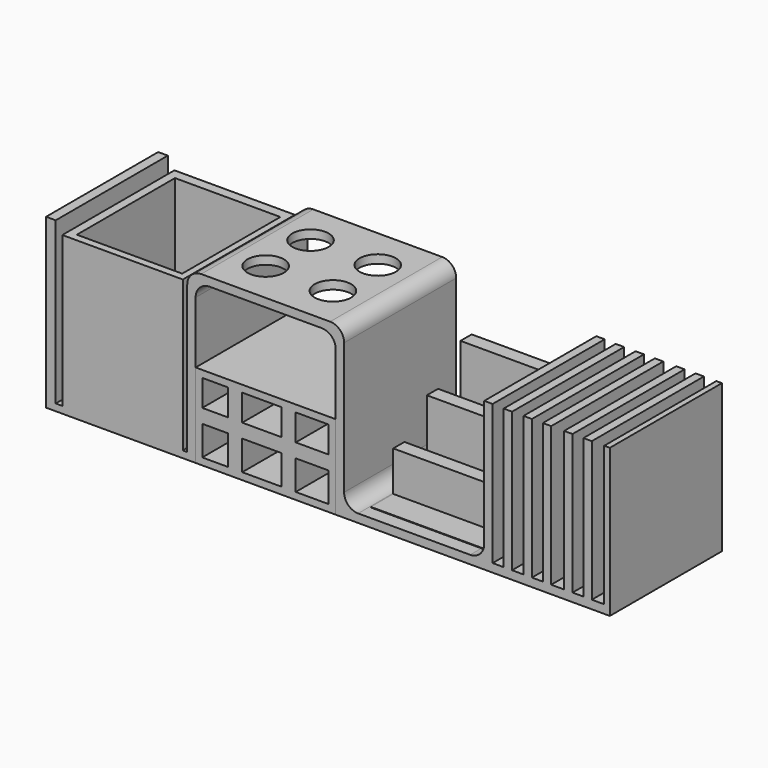
from build123d import *

# Parameters (mm, degrees)
F0_W      = 2
F0_H      = 49.8195460532
F0_W_2    = 3
F1_DEPTH  = 50
F4_W      = 40
F4_H      = 15
F5_DEPTH  = 36.1
F6_W      = 40
F6_H      = 10
F7_DEPTH  = 35.5
F8_W      = 40
F8_H      = 15
F9_DEPTH  = 25.1
F10_W     = 40
F10_H     = 10
F11_DEPTH = 24.8
F12_W     = 40
F12_H     = 15
F13_DEPTH = 14.5
F14_W     = 40
F14_H     = 10
F15_DEPTH = 14.3
F16_R     = 5
F3_W      = 50
F3_H      = 50
F17_DEPTH = 30
F18_T     = -2.5
F2_R      = 6.5
F19_DEPTH = 13.9
F20_W     = 43
F20_H     = 50
F21_DEPTH = 53.7
F22_W     = 37.6056898385
F22_H     = 43.7766639516
F23_DEPTH = 51.1
F24_W     = 9.2634954209
F24_H     = 5.0000008196
F24_W_2   = 5.0000008196
F24_H_2   = 9.4318167865
F24_W_3   = 14.0909086913
F24_H_3   = 10.5681823939
F24_W_4   = 5.0000026822
F24_W_5   = 11.6455923861
F25_DEPTH = 47.5


with BuildPart() as f1:
    # F0 (on Front) → F1 (new body)
    with BuildSketch(Plane.XZ):
        Polygon((4.5763543636, 0), (4.5763543636, 57), (54.5763543636, 57), (54.5763543636, 0), (107.5763543636, 0), (107.5763543636, 3), (57.5763543636, 3), (57.5763543636, 60), (1.5763543636, 60), (1.5763543636, 2.4467778858), (-45.3553423285, 2.4467778858), (-45.3553423285, 60), (-48.798955977, 60), (-48.798955977, 0), (-45.3553423285, 0), (1.5763543636, 0), align=None)
        Polygon((107.5763543636, 3), (107.5763543636, 0), (110.5763543636, 0), (152.4111737013, 0), (152.4111737013, 3.0127370264), (150.4111737013, 3.0127370264), (145.9802030325, 3.0127370264), (142.9802030325, 3.0127370264), (139.0929906368, 3.0127370264), (136.0929906368, 3.0127370264), (131.4807920456, 3.0127370264), (128.4807920456, 3.0127370264), (124.5935647488, 3.0127370264), (121.5935647488, 3.0127370264), (117.5098730922, 3.0127370264), (114.5098730922, 3.0127370264), (110.5763543636, 3.0127370264), (110.5763543636, 53), (107.5763543636, 53), align=None)
        with Locations((151.4111737013, 27.922510053)):
            Rectangle(F0_W, F0_H)
        with Locations((144.4802030325, 27.922510053)):
            Rectangle(F0_W_2, F0_H)
        with Locations((116.0098730922, 27.922510053)):
            Rectangle(F0_W_2, F0_H)
        with Locations((137.5929906368, 27.922510053)):
            Rectangle(F0_W_2, F0_H)
        with Locations((123.0935647488, 27.922510053)):
            Rectangle(F0_W_2, F0_H)
        with Locations((129.9807920456, 27.922510053)):
            Rectangle(F0_W_2, F0_H)
    extrude(amount=F1_DEPTH)

    # F4 (on face) → F5 (join)
    with BuildSketch(Plane.XY.offset(3)):
        with Locations((83.0988776684, -7.5)):
            Rectangle(F4_W, F4_H)
    extrude(amount=F5_DEPTH)

    # F6 (on face) → F7 (cut)
    with BuildSketch(Plane.XY.offset(39.1)):
        with Locations((83.0988776684, -10)):
            Rectangle(F6_W, F6_H)
    extrude(amount=-F7_DEPTH, mode=Mode.SUBTRACT)

    # F8 (on face) → F9 (join)
    with BuildSketch(Plane.XY.offset(3)):
        with Locations((83.0988776684, -22.5)):
            Rectangle(F8_W, F8_H)
    extrude(amount=F9_DEPTH)

    # F10 (on face) → F11 (cut)
    with BuildSketch(Plane.XY.offset(28.1)):
        with Locations((83.0988776684, -25)):
            Rectangle(F10_W, F10_H)
    extrude(amount=-F11_DEPTH, mode=Mode.SUBTRACT)

    # F12 (on face) → F13 (join)
    with BuildSketch(Plane.XY.offset(3)):
        with Locations((83.0988776684, -37.5)):
            Rectangle(F12_W, F12_H)
    extrude(amount=F13_DEPTH)

    # F14 (on face) → F15 (cut)
    with BuildSketch(Plane.XY.offset(17.5)):
        with Locations((83.0988776684, -40)):
            Rectangle(F14_W, F14_H)
    extrude(amount=-F15_DEPTH, mode=Mode.SUBTRACT)

    # F16
    f16_edges = [f1.edges().sort_by_distance(p)[0] for p in [
        (57.576354, -25, 60),
        (54.576354, -25, 57),
        (4.576354, -25, 57),
        (57.576354, -25, 3),
        (107.576354, -25, 3),
        (1.576354, -25, 60),
    ]]
    fillet(f16_edges, radius=F16_R)

    # F2 (on face) + F10 (on face) → F19 (cut)
    with BuildSketch(Plane.XY.offset(60)):
        with Locations((17.5763543636, -15)):
            Circle(F2_R)
        with Locations((41.5763543636, -15)):
            Circle(F2_R)
        with Locations((17.5763543636, -35)):
            Circle(F2_R)
        with Locations((41.5763543636, -35)):
            Circle(F2_R)
    with BuildSketch(Plane.XY.offset(28.1)):
        with Locations((83.0988776684, -25)):
            Rectangle(F10_W, F10_H)
    extrude(amount=-F19_DEPTH, mode=Mode.SUBTRACT)

    # F20 (on face) → F21 (join)
    with BuildSketch(Plane.XY.offset(2.4467778858)):
        with Locations((-21.5, -25)):
            Rectangle(F20_W, F20_H)
    extrude(amount=F21_DEPTH)

    # F22 (on face) → F23 (cut)
    with BuildSketch(Plane.XY.offset(56.1467778858)):
        with Locations((-21.1496120319, -25.4395254888)):
            Rectangle(F22_W, F22_H)
    extrude(amount=-F23_DEPTH, mode=Mode.SUBTRACT)


with BuildPart() as f17:
    # F3 (on Top) → F17 (new body)
    with BuildSketch(Plane.XY):
        with Locations((29.4420910721, -25)):
            Rectangle(F3_W, F3_H)
    extrude(amount=F17_DEPTH)

    # F18
    f18_openings = [f17.faces().sort_by_distance(p)[0] for p in [
        (29.442091, -50, 15),
    ]]
    offset(amount=F18_T, openings=f18_openings)

    # F24 (on face) → F25 (join)
    with BuildSketch(Plane.XZ.offset(2.5)):
        with Locations((11.5738387826, 15.5681828037)):
            Rectangle(F24_W, F24_H)
        with Locations((18.7055869028, 22.7840916067)):
            Rectangle(F24_W_2, F24_H_2)
        with Locations((18.7055869028, 15.5681828037)):
            Rectangle(F24_W_2, F24_H)
        with Locations((28.2510416582, 15.5681828037)):
            Rectangle(F24_W_3, F24_H)
        with Locations((18.7055869028, 7.784091197)):
            Rectangle(F24_W_2, F24_H_3)
        with Locations((37.796497345, 22.7840916067)):
            Rectangle(F24_W_4, F24_H_2)
        with Locations((37.796497345, 15.5681828037)):
            Rectangle(F24_W_4, F24_H)
        with Locations((46.1192948791, 15.5681828037)):
            Rectangle(F24_W_5, F24_H)
        with Locations((37.796497345, 7.784091197)):
            Rectangle(F24_W_4, F24_H_3)
    extrude(amount=F25_DEPTH)


solid = Compound([f1.part, f17.part])
